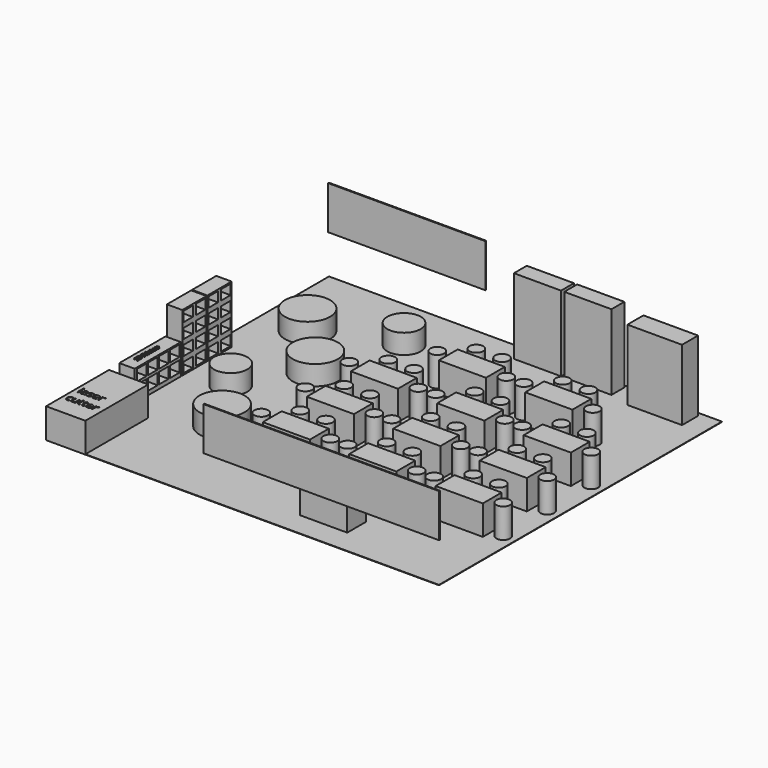
from build123d import *

# Parameters (mm, degrees)
F0_W          = 10000
F0_H          = 9000
F1_DEPTH      = 10
F2_W          = 1200
F2_H          = 600
F2_R          = 175
F3_DEPTH      = 750
F5_W          = 6000
F5_H          = 1100
F6_DEPTH      = 25
F8_W          = 1200
F8_H          = 410
F9_DEPTH      = 1920
F10_W         = 1390
F10_H         = 510
F11_DEPTH     = 1800
F12_W         = 4000
F12_H         = 1100
F13_DEPTH     = 25
F15_W         = 770
F15_H         = 1470
F15_W_2       = 298.1355935335
F15_H_2       = 253.6377906799
F16_DEPTH     = 390
F17_R         = 575
F17_R_2       = 425
F18_DEPTH     = 500
F19_W         = 1000
F19_H         = 2000
F19_W_2       = 23.0397869153
F19_H_2       = 215.8814716164
F20_DEPTH     = 750
F21_W         = 311.8368387222
F21_H         = 282.1381092072
F22_DEPTH     = 390
F23_TEXT_SIZE = 138.8888888889
F24_DEPTH     = 25


# Not quite as in the source:
# - Text() gives the source's letters only with a copy of the font that has no kerning and outlines rounded to 1/6400 em; it was checked with that copy


with BuildPart() as f1:
    # F0 (on Top) → F1 (new body)
    with BuildSketch(Plane.XY):
        Rectangle(F0_W, F0_H)
    extrude(amount=-F1_DEPTH)

    # F2 (on Top) → F3 (join)
    with BuildSketch(Plane.XY):
        with Locations((1572.2411870956, -3585.0810220754)):
            Rectangle(F2_W, F2_H)
        with Locations((3789.9301052094, -2043.914437294)):
            Rectangle(F2_W, F2_H)
        with Locations((2914.3524169922, -2047.3065376282)):
            Circle(F2_R)
        with Locations((4108.0131530762, -1479.732632637)):
            Circle(F2_R)
        with Locations((3458.5213661194, -1485.5839014053)):
            Circle(F2_R)
        with Locations((4681.4386844635, -2059.0091347694)):
            Circle(F2_R)
        with Locations((2914.3524169922, -647.3065376282)):
            Circle(F2_R)
        with Locations((4681.4386844635, -659.0091347694)):
            Circle(F2_R)
        with Locations((3789.9301052094, -643.914437294)):
            Rectangle(F2_W, F2_H)
        with Locations((3458.5213661194, -85.5839014053)):
            Circle(F2_R)
        with Locations((4108.0131530762, -79.732632637)):
            Circle(F2_R)
        with Locations((2914.3524169922, 752.6934623718)):
            Circle(F2_R)
        with Locations((4681.4386844635, 740.9908652306)):
            Circle(F2_R)
        with Locations((3789.9301052094, 756.085562706)):
            Rectangle(F2_W, F2_H)
        with Locations((3458.5213661194, 1314.4160985947)):
            Circle(F2_R)
        with Locations((4108.0131530762, 1320.267367363)):
            Circle(F2_R)
        with Locations((714.3524169922, -2047.3065376282)):
            Circle(F2_R)
        with Locations((2481.4386844635, -2059.0091347694)):
            Circle(F2_R)
        with Locations((1589.9301052094, -2043.914437294)):
            Rectangle(F2_W, F2_H)
        with Locations((1258.5213661194, -1485.5839014053)):
            Circle(F2_R)
        with Locations((1908.0131530762, -1479.732632637)):
            Circle(F2_R)
        with Locations((714.3524169922, -647.3065376282)):
            Circle(F2_R)
        with Locations((2481.4386844635, -659.0091347694)):
            Circle(F2_R)
        with Locations((1589.9301052094, -643.914437294)):
            Rectangle(F2_W, F2_H)
        with Locations((1258.5213661194, -85.5839014053)):
            Circle(F2_R)
        with Locations((1908.0131530762, -79.732632637)):
            Circle(F2_R)
        with Locations((714.3524169922, 752.6934623718)):
            Circle(F2_R)
        with Locations((2481.4386844635, 740.9908652306)):
            Circle(F2_R)
        with Locations((1589.9301052094, 756.085562706)):
            Rectangle(F2_W, F2_H)
        with Locations((1258.5213661194, 1314.4160985947)):
            Circle(F2_R)
        with Locations((1908.0131530762, 1320.267367363)):
            Circle(F2_R)
        with Locations((-1485.6475830078, -2047.3065376282)):
            Circle(F2_R)
        with Locations((281.4386844635, -2059.0091347694)):
            Circle(F2_R)
        with Locations((-610.0698947906, -2043.914437294)):
            Rectangle(F2_W, F2_H)
        with Locations((-941.4786338806, -1485.5839014053)):
            Circle(F2_R)
        with Locations((-291.9868469238, -1479.732632637)):
            Circle(F2_R)
        with Locations((-1485.6475830078, -647.3065376282)):
            Circle(F2_R)
        with Locations((281.4386844635, -659.0091347694)):
            Circle(F2_R)
        with Locations((-610.0698947906, -643.914437294)):
            Rectangle(F2_W, F2_H)
        with Locations((-941.4786338806, -85.5839014053)):
            Circle(F2_R)
        with Locations((-291.9868469238, -79.732632637)):
            Circle(F2_R)
        with Locations((-1485.6475830078, 752.6934623718)):
            Circle(F2_R)
        with Locations((281.4386844635, 740.9908652306)):
            Circle(F2_R)
        with Locations((-610.0698947906, 756.085562706)):
            Rectangle(F2_W, F2_H)
        with Locations((-941.4786338806, 1314.4160985947)):
            Circle(F2_R)
        with Locations((-291.9868469238, 1320.267367363)):
            Circle(F2_R)
        with Locations((1784.7433149815, 2214.4345091656)):
            Circle(F2_R)
        with Locations((3551.8295824528, 2202.7319120243)):
            Circle(F2_R)
        with Locations((2660.3210031986, 2217.8266094998)):
            Rectangle(F2_W, F2_H)
        with Locations((2328.9122641087, 2776.1571453884)):
            Circle(F2_R)
        with Locations((2978.4040510654, 2782.0084141567)):
            Circle(F2_R)
        with Locations((-415.2566850185, 2214.4345091656)):
            Circle(F2_R)
        with Locations((1351.8295824528, 2202.7319120243)):
            Circle(F2_R)
        with Locations((460.3210031986, 2217.8266094998)):
            Rectangle(F2_W, F2_H)
        with Locations((128.9122641087, 2776.1571453884)):
            Circle(F2_R)
        with Locations((778.4040510654, 2782.0084141567)):
            Circle(F2_R)
    extrude(amount=F3_DEPTH)

    # F8 (on Top) → F9 (join)
    with BuildSketch(Plane.XY):
        with Locations((686.8221908808, 4228.9738616641)):
            Rectangle(F8_W, F8_H)
        with Locations((1969.4395661354, 4228.5027503967)):
            Rectangle(F8_W, F8_H)
    extrude(amount=F9_DEPTH)

    # F10 (on Top) → F11 (join)
    with BuildSketch(Plane.XY):
        with Locations((3781.6548347473, 4139.8178529011)):
            Rectangle(F10_W, F10_H)
    extrude(amount=F11_DEPTH)

    # F15 (on offset) → F16 (join)
    with BuildSketch(Plane.YZ.offset(-5000)):
        with Locations((529.4889600399, 735)):
            Rectangle(F15_W, F15_H)
        with Locations((329.677836597, 165.8990240097)):
            Rectangle(F15_W_2, F15_H_2, mode=Mode.SUBTRACT)
        with Locations((729.677836597, 165.8990240097)):
            Rectangle(F15_W_2, F15_H_2, mode=Mode.SUBTRACT)
        with Locations((329.677836597, 545.8990240097)):
            Rectangle(F15_W_2, F15_H_2, mode=Mode.SUBTRACT)
        with Locations((729.677836597, 545.8990240097)):
            Rectangle(F15_W_2, F15_H_2, mode=Mode.SUBTRACT)
        with Locations((329.677836597, 925.8990240097)):
            Rectangle(F15_W_2, F15_H_2, mode=Mode.SUBTRACT)
        with Locations((729.677836597, 925.8990240097)):
            Rectangle(F15_W_2, F15_H_2, mode=Mode.SUBTRACT)
        with Locations((329.677836597, 1305.8990240097)):
            Rectangle(F15_W_2, F15_H_2, mode=Mode.SUBTRACT)
        with Locations((729.677836597, 1305.8990240097)):
            Rectangle(F15_W_2, F15_H_2, mode=Mode.SUBTRACT)
        with Locations((-270.5110399601, 735)):
            Rectangle(F15_W, F15_H)
        with Locations((-470.322163403, 165.8990240097)):
            Rectangle(F15_W_2, F15_H_2, mode=Mode.SUBTRACT)
        with Locations((-70.322163403, 165.8990240097)):
            Rectangle(F15_W_2, F15_H_2, mode=Mode.SUBTRACT)
        with Locations((-470.322163403, 545.8990240097)):
            Rectangle(F15_W_2, F15_H_2, mode=Mode.SUBTRACT)
        with Locations((-70.322163403, 545.8990240097)):
            Rectangle(F15_W_2, F15_H_2, mode=Mode.SUBTRACT)
        with Locations((-470.322163403, 925.8990240097)):
            Rectangle(F15_W_2, F15_H_2, mode=Mode.SUBTRACT)
        with Locations((-70.322163403, 925.8990240097)):
            Rectangle(F15_W_2, F15_H_2, mode=Mode.SUBTRACT)
        with Locations((-470.322163403, 1305.8990240097)):
            Rectangle(F15_W_2, F15_H_2, mode=Mode.SUBTRACT)
        with Locations((-70.322163403, 1305.8990240097)):
            Rectangle(F15_W_2, F15_H_2, mode=Mode.SUBTRACT)
    extrude(amount=F16_DEPTH)

    # F17 (on Top) → F18 (join)
    with BuildSketch(Plane.XY):
        with Locations((-3872.6794719696, 2408.0123901367)):
            Circle(F17_R)
        with Locations((-2614.8862838745, 1084.0193033218)):
            Circle(F17_R)
        with Locations((-2631.4361095428, -1861.8651628494)):
            Circle(F17_R)
        with Locations((-3591.3310050964, -388.9229595661)):
            Circle(F17_R_2)
        with Locations((-1985.9894514084, 3119.6584701538)):
            Circle(F17_R_2)
    extrude(amount=F18_DEPTH)

    # F19 (on face) → F20 (join)
    with BuildSketch(Plane.XY):
        with Locations((-4500, -3500)):
            Rectangle(F19_W, F19_H)
        with BuildLine():
            add(Edge.make_bspline(
                [(-4797.4227787473, -4022.5041243538), (-4812.6494587318, -4030.4504092436), (-4835.8224236061, -4030.4504092436)],
                knots=[0, 0, 0, 1, 1, 1], degree=2))
            add(Edge.make_bspline(
                [(-4835.8224236061, -4030.4504092436), (-4868.8505574499, -4030.4504092436), (-4886.9627598804, -4010.1185741624)],
                knots=[0, 0, 0, 1, 1, 1], degree=2))
            add(Edge.make_bspline(
                [(-4886.9627598804, -4010.1185741624), (-4905.0749623109, -3989.7867390811), (-4905.0749623109, -3952.5856958537)],
                knots=[0, 0, 0, 1, 1, 1], degree=2))
            add(Edge.make_bspline(
                [(-4905.0749623109, -3952.5856958537), (-4905.0749623109, -3914.452406913), (-4886.6742076358, -3893.6322526486)],
                knots=[0, 0, 0, 1, 1, 1], degree=2))
            add(Edge.make_bspline(
                [(-4886.6742076358, -3893.6322526486), (-4868.2734529607, -3872.8120983841), (-4834.3130734035, -3872.8120983841)],
                knots=[0, 0, 0, 1, 1, 1], degree=2))
            add(Edge.make_bspline(
                [(-4834.3130734035, -3872.8120983841), (-4823.3480881086, -3872.8120983841), (-4812.3831028137, -3875.1871053204)],
                knots=[0, 0, 0, 1, 1, 1], degree=2))
            add(Edge.make_bspline(
                [(-4812.3831028137, -3875.1871053204), (-4801.4181175187, -3877.5621122568), (-4795.2031460965, -3880.7583832739)],
                knots=[0, 0, 0, 1, 1, 1], degree=2))
            Line((-4795.2031460965, -3880.7583832739), (-4802.2615779261, -3900.291150601))
            add(Edge.make_bspline(
                [(-4802.2615779261, -3900.291150601), (-4809.8971142448, -3897.2280575429), (-4818.908822807, -3895.2303881571)],
                knots=[0, 0, 0, 1, 1, 1], degree=2))
            add(Edge.make_bspline(
                [(-4818.908822807, -3895.2303881571), (-4827.9205313693, -3893.2327187714), (-4834.8457852397, -3893.2327187714)],
                knots=[0, 0, 0, 1, 1, 1], degree=2))
            add(Edge.make_bspline(
                [(-4834.8457852397, -3893.2327187714), (-4881.1917149884, -3893.2327187714), (-4881.1917149884, -3952.3193399356)],
                knots=[0, 0, 0, 1, 1, 1], degree=2))
            add(Edge.make_bspline(
                [(-4881.1917149884, -3952.3193399356), (-4881.1917149884, -3980.3311039887), (-4869.8937847958, -3995.3136243815)],
                knots=[0, 0, 0, 1, 1, 1], degree=2))
            add(Edge.make_bspline(
                [(-4869.8937847958, -3995.3136243815), (-4858.5958546033, -4010.2961447744), (-4836.3995280953, -4010.2961447744)],
                knots=[0, 0, 0, 1, 1, 1], degree=2))
            add(Edge.make_bspline(
                [(-4836.3995280953, -4010.2961447744), (-4817.3994726045, -4010.2961447744), (-4797.4227787473, -4002.1278966195)],
                knots=[0, 0, 0, 1, 1, 1], degree=2))
            Line((-4797.4227787473, -4002.1278966195), (-4797.4227787473, -4022.5041243538))
        make_face(mode=Mode.SUBTRACT)
        with BuildLine():
            Line((-4762.974080007, -3875.6088355241), (-4739.6679371736, -3875.6088355241))
            Line((-4739.6679371736, -3875.6088355241), (-4739.6679371736, -3974.2493105255))
            add(Edge.make_bspline(
                [(-4739.6679371736, -3974.2493105255), (-4739.6679371736, -3992.8498321392), (-4731.2111367741, -4001.9947186604)],
                knots=[0, 0, 0, 1, 1, 1], degree=2))
            add(Edge.make_bspline(
                [(-4731.2111367741, -4001.9947186604), (-4722.7543363745, -4011.1396051817), (-4704.7309192501, -4011.1396051817)],
                knots=[0, 0, 0, 1, 1, 1], degree=2))
            add(Edge.make_bspline(
                [(-4704.7309192501, -4011.1396051817), (-4680.8476719275, -4011.1396051817), (-4669.8382939795, -3998.1103615215)],
                knots=[0, 0, 0, 1, 1, 1], degree=2))
            add(Edge.make_bspline(
                [(-4669.8382939795, -3998.1103615215), (-4658.8289160316, -3985.0811178614), (-4658.8289160316, -3955.5156109528)],
                knots=[0, 0, 0, 1, 1, 1], degree=2))
            Line((-4658.8289160316, -3955.5156109528), (-4658.8289160316, -3875.6088355241))
            Line((-4658.8289160316, -3875.6088355241), (-4635.7891291163, -3875.6088355241))
            Line((-4635.7891291163, -3875.6088355241), (-4635.7891291163, -4027.6536721036))
            Line((-4635.7891291163, -4027.6536721036), (-4654.7891846071, -4027.6536721036))
            Line((-4654.7891846071, -4027.6536721036), (-4658.1186335833, -4007.2774443693))
            Line((-4658.1186335833, -4007.2774443693), (-4659.3616278678, -4007.2774443693))
            add(Edge.make_bspline(
                [(-4659.3616278678, -4007.2774443693), (-4666.4200596973, -4018.5087855824), (-4678.9831805008, -4024.479597413)],
                knots=[0, 0, 0, 1, 1, 1], degree=2))
            add(Edge.make_bspline(
                [(-4678.9831805008, -4024.479597413), (-4691.5463013043, -4030.4504092436), (-4707.6608343491, -4030.4504092436)],
                knots=[0, 0, 0, 1, 1, 1], degree=2))
            add(Edge.make_bspline(
                [(-4707.6608343491, -4030.4504092436), (-4735.4062424841, -4030.4504092436), (-4749.1901612455, -4017.2657912979)],
                knots=[0, 0, 0, 1, 1, 1], degree=2))
            add(Edge.make_bspline(
                [(-4749.1901612455, -4017.2657912979), (-4762.974080007, -4004.0811733522), (-4762.974080007, -3975.0927709328)],
                knots=[0, 0, 0, 1, 1, 1], degree=2))
            Line((-4762.974080007, -3975.0927709328), (-4762.974080007, -3875.6088355241))
        make_face(mode=Mode.SUBTRACT)
        with BuildLine():
            add(Edge.make_bspline(
                [(-4295.8745849734, -4028.1419912868), (-4306.7507849623, -4030.4504092436), (-4322.1550355588, -4030.4504092436)],
                knots=[0, 0, 0, 1, 1, 1], degree=2))
            add(Edge.make_bspline(
                [(-4322.1550355588, -4030.4504092436), (-4355.8490591979, -4030.4504092436), (-4375.3596301984, -4009.8966108973)],
                knots=[0, 0, 0, 1, 1, 1], degree=2))
            add(Edge.make_bspline(
                [(-4375.3596301984, -4009.8966108973), (-4394.8702011989, -3989.3428125509), (-4394.8702011989, -3952.8964444248)],
                knots=[0, 0, 0, 1, 1, 1], degree=2))
            add(Edge.make_bspline(
                [(-4394.8702011989, -3952.8964444248), (-4394.8702011989, -3916.0949350746), (-4376.7579987684, -3894.4535167294)],
                knots=[0, 0, 0, 1, 1, 1], degree=2))
            add(Edge.make_bspline(
                [(-4376.7579987684, -3894.4535167294), (-4358.6457963379, -3872.8120983841), (-4328.1036510629, -3872.8120983841)],
                knots=[0, 0, 0, 1, 1, 1], degree=2))
            add(Edge.make_bspline(
                [(-4328.1036510629, -3872.8120983841), (-4299.5591751737, -3872.8120983841), (-4282.9119302927, -3891.6123869363)],
                knots=[0, 0, 0, 1, 1, 1], degree=2))
            add(Edge.make_bspline(
                [(-4282.9119302927, -3891.6123869363), (-4266.2646854118, -3910.4126754886), (-4266.2646854118, -3941.2211766816)],
                knots=[0, 0, 0, 1, 1, 1], degree=2))
            Line((-4266.2646854118, -3941.2211766816), (-4266.2646854118, -3955.7819668709))
            Line((-4266.2646854118, -3955.7819668709), (-4370.9869538763, -3955.7819668709))
            add(Edge.make_bspline(
                [(-4370.9869538763, -3955.7819668709), (-4370.2766714281, -3982.5507366395), (-4357.4471947065, -3996.4234407069)],
                knots=[0, 0, 0, 1, 1, 1], degree=2))
            add(Edge.make_bspline(
                [(-4357.4471947065, -3996.4234407069), (-4344.6177179849, -4010.2961447744), (-4321.3115751515, -4010.2961447744)],
                knots=[0, 0, 0, 1, 1, 1], degree=2))
            add(Edge.make_bspline(
                [(-4321.3115751515, -4010.2961447744), (-4296.7624380337, -4010.2961447744), (-4272.7904054051, -4000.0414419277)],
                knots=[0, 0, 0, 1, 1, 1], degree=2))
            Line((-4272.7904054051, -4000.0414419277), (-4272.7904054051, -4020.5952402741))
            add(Edge.make_bspline(
                [(-4272.7904054051, -4020.5952402741), (-4284.9983849845, -4025.83357333), (-4295.8745849734, -4028.1419912868)],
                knots=[0, 0, 0, 1, 1, 1], degree=2))
        make_face(mode=Mode.SUBTRACT)
        with BuildLine():
            add(Edge.make_bspline(
                [(-4183.8275287612, -3880.8693649065), (-4171.8859050999, -3872.8120983841), (-4157.5914708288, -3872.8120983841)],
                knots=[0, 0, 0, 1, 1, 1], degree=2))
            add(Edge.make_bspline(
                [(-4157.5914708288, -3872.8120983841), (-4147.4699459411, -3872.8120983841), (-4139.4348757453, -3874.4990191987)],
                knots=[0, 0, 0, 1, 1, 1], degree=2))
            Line((-4139.4348757453, -3874.4990191987), (-4142.6311467624, -3895.8518852994))
            add(Edge.make_bspline(
                [(-4142.6311467624, -3895.8518852994), (-4152.0423892018, -3893.7654306076), (-4159.2783916434, -3893.7654306076)],
                knots=[0, 0, 0, 1, 1, 1], degree=2))
            add(Edge.make_bspline(
                [(-4159.2783916434, -3893.7654306076), (-4177.745735298, -3893.7654306076), (-4190.8415679377, -3908.7479510005)],
                knots=[0, 0, 0, 1, 1, 1], degree=2))
            add(Edge.make_bspline(
                [(-4190.8415679377, -3908.7479510005), (-4203.9374005774, -3923.7304713934), (-4203.9374005774, -3946.0599758604)],
                knots=[0, 0, 0, 1, 1, 1], degree=2))
            Line((-4203.9374005774, -3946.0599758604), (-4203.9374005774, -4027.6536721036))
            Line((-4203.9374005774, -4027.6536721036), (-4226.9771874927, -4027.6536721036))
            Line((-4226.9771874927, -4027.6536721036), (-4226.9771874927, -3875.6088355241))
            Line((-4226.9771874927, -3875.6088355241), (-4207.9771320019, -3875.6088355241))
            Line((-4207.9771320019, -3875.6088355241), (-4205.3135728209, -3903.7537775362))
            Line((-4205.3135728209, -3903.7537775362), (-4204.2037564955, -3903.7537775362))
            add(Edge.make_bspline(
                [(-4204.2037564955, -3903.7537775362), (-4195.7691524225, -3888.9266314289), (-4183.8275287612, -3880.8693649065)],
                knots=[0, 0, 0, 1, 1, 1], degree=2))
        make_face(mode=Mode.SUBTRACT)
        with BuildLine():
            add(Edge.make_bspline(
                [(-4555.7491757286, -4004.0589770257), (-4549.2234557353, -4011.4059610998), (-4537.8589365632, -4011.4059610998)],
                knots=[0, 0, 0, 1, 1, 1], degree=2))
            add(Edge.make_bspline(
                [(-4537.8589365632, -4011.4059610998), (-4531.732750447, -4011.4059610998), (-4526.050490861, -4010.5181080395)],
                knots=[0, 0, 0, 1, 1, 1], degree=2))
            add(Edge.make_bspline(
                [(-4526.050490861, -4010.5181080395), (-4520.3682312749, -4009.6302549792), (-4517.0387822987, -4008.6536166128)],
                knots=[0, 0, 0, 1, 1, 1], degree=2))
            Line((-4517.0387822987, -4008.6536166128), (-4517.0387822987, -4026.2774998602))
            add(Edge.make_bspline(
                [(-4517.0387822987, -4026.2774998602), (-4520.7677651521, -4028.0532059808), (-4528.0481602467, -4029.2518076122)],
                knots=[0, 0, 0, 1, 1, 1], degree=2))
            add(Edge.make_bspline(
                [(-4528.0481602467, -4029.2518076122), (-4535.3285553413, -4030.4504092436), (-4541.1883855394, -4030.4504092436)],
                knots=[0, 0, 0, 1, 1, 1], degree=2))
            add(Edge.make_bspline(
                [(-4541.1883855394, -4030.4504092436), (-4585.2702899842, -4030.4504092436), (-4585.2702899842, -3983.971301536)],
                knots=[0, 0, 0, 1, 1, 1], degree=2))
            Line((-4585.2702899842, -3983.971301536), (-4585.2702899842, -3893.4990746895))
            Line((-4585.2702899842, -3893.4990746895), (-4607.067082615, -3893.4990746895))
            Line((-4607.067082615, -3893.4990746895), (-4607.067082615, -3882.4009114355))
            Line((-4607.067082615, -3882.4009114355), (-4585.2702899842, -3872.8120983841))
            Line((-4585.2702899842, -3872.8120983841), (-4575.5926916267, -3840.3610690295))
            Line((-4575.5926916267, -3840.3610690295), (-4562.274895722, -3840.3610690295))
            Line((-4562.274895722, -3840.3610690295), (-4562.274895722, -3875.6088355241))
            Line((-4562.274895722, -3875.6088355241), (-4518.1485986241, -3875.6088355241))
            Line((-4518.1485986241, -3875.6088355241), (-4518.1485986241, -3893.4990746895))
            Line((-4518.1485986241, -3893.4990746895), (-4562.274895722, -3893.4990746895))
            Line((-4562.274895722, -3893.4990746895), (-4562.274895722, -3982.9946631696))
            add(Edge.make_bspline(
                [(-4562.274895722, -3982.9946631696), (-4562.274895722, -3996.7119929515), (-4555.7491757286, -4004.0589770257)],
                knots=[0, 0, 0, 1, 1, 1], degree=2))
        make_face(mode=Mode.SUBTRACT)
        with BuildLine():
            add(Edge.make_bspline(
                [(-4455.4661725656, -4004.0589770257), (-4448.9404525723, -4011.4059610998), (-4437.5759334002, -4011.4059610998)],
                knots=[0, 0, 0, 1, 1, 1], degree=2))
            add(Edge.make_bspline(
                [(-4437.5759334002, -4011.4059610998), (-4431.449747284, -4011.4059610998), (-4425.767487698, -4010.5181080395)],
                knots=[0, 0, 0, 1, 1, 1], degree=2))
            add(Edge.make_bspline(
                [(-4425.767487698, -4010.5181080395), (-4420.0852281119, -4009.6302549792), (-4416.7557791358, -4008.6536166128)],
                knots=[0, 0, 0, 1, 1, 1], degree=2))
            Line((-4416.7557791358, -4008.6536166128), (-4416.7557791358, -4026.2774998602))
            add(Edge.make_bspline(
                [(-4416.7557791358, -4026.2774998602), (-4420.4847619891, -4028.0532059808), (-4427.7651570837, -4029.2518076122)],
                knots=[0, 0, 0, 1, 1, 1], degree=2))
            add(Edge.make_bspline(
                [(-4427.7651570837, -4029.2518076122), (-4435.0455521783, -4030.4504092436), (-4440.9053823764, -4030.4504092436)],
                knots=[0, 0, 0, 1, 1, 1], degree=2))
            add(Edge.make_bspline(
                [(-4440.9053823764, -4030.4504092436), (-4484.9872868212, -4030.4504092436), (-4484.9872868212, -3983.971301536)],
                knots=[0, 0, 0, 1, 1, 1], degree=2))
            Line((-4484.9872868212, -3983.971301536), (-4484.9872868212, -3893.4990746895))
            Line((-4484.9872868212, -3893.4990746895), (-4506.784079452, -3893.4990746895))
            Line((-4506.784079452, -3893.4990746895), (-4506.784079452, -3882.4009114355))
            Line((-4506.784079452, -3882.4009114355), (-4484.9872868212, -3872.8120983841))
            Line((-4484.9872868212, -3872.8120983841), (-4475.3096884638, -3840.3610690295))
            Line((-4475.3096884638, -3840.3610690295), (-4461.991892559, -3840.3610690295))
            Line((-4461.991892559, -3840.3610690295), (-4461.991892559, -3875.6088355241))
            Line((-4461.991892559, -3875.6088355241), (-4417.8655954611, -3875.6088355241))
            Line((-4417.8655954611, -3875.6088355241), (-4417.8655954611, -3893.4990746895))
            Line((-4417.8655954611, -3893.4990746895), (-4461.991892559, -3893.4990746895))
            Line((-4461.991892559, -3893.4990746895), (-4461.991892559, -3982.9946631696))
            add(Edge.make_bspline(
                [(-4461.991892559, -3982.9946631696), (-4461.991892559, -3996.7119929515), (-4455.4661725656, -4004.0589770257)],
                knots=[0, 0, 0, 1, 1, 1], degree=2))
        make_face(mode=Mode.SUBTRACT)
        with Locations((-4885.0760721273, -3533.3192844448)):
            Rectangle(F19_W_2, F19_H_2, mode=Mode.SUBTRACT)
        with BuildLine():
            Line((-4714.1421616894, -3641.260020253), (-4731.2333331006, -3641.260020253))
            Line((-4731.2333331006, -3641.260020253), (-4735.8057763612, -3619.5964055813))
            Line((-4735.8057763612, -3619.5964055813), (-4736.9155926866, -3619.5964055813))
            add(Edge.make_bspline(
                [(-4736.9155926866, -3619.5964055813), (-4748.2801118587, -3633.8908398524), (-4759.5780420512, -3638.9737986227)],
                knots=[0, 0, 0, 1, 1, 1], degree=2))
            add(Edge.make_bspline(
                [(-4759.5780420512, -3638.9737986227), (-4770.8759722438, -3644.056757393), (-4787.8339656959, -3644.056757393)],
                knots=[0, 0, 0, 1, 1, 1], degree=2))
            add(Edge.make_bspline(
                [(-4787.8339656959, -3644.056757393), (-4810.429826081, -3644.056757393), (-4823.2593028026, -3632.3814896498)],
                knots=[0, 0, 0, 1, 1, 1], degree=2))
            add(Edge.make_bspline(
                [(-4823.2593028026, -3632.3814896498), (-4836.0887795242, -3620.7062219067), (-4836.0887795242, -3599.2201778469)],
                knots=[0, 0, 0, 1, 1, 1], degree=2))
            add(Edge.make_bspline(
                [(-4836.0887795242, -3599.2201778469), (-4836.0887795242, -3553.1849966694), (-4762.4413681708, -3550.9653640186)],
                knots=[0, 0, 0, 1, 1, 1], degree=2))
            Line((-4762.4413681708, -3550.9653640186), (-4736.6492367685, -3550.1219036113))
            Line((-4736.6492367685, -3550.1219036113), (-4736.6492367685, -3540.6662685189))
            add(Edge.make_bspline(
                [(-4736.6492367685, -3540.6662685189), (-4736.6492367685, -3522.7760293535), (-4744.3291657403, -3514.2526399745)],
                knots=[0, 0, 0, 1, 1, 1], degree=2))
            add(Edge.make_bspline(
                [(-4744.3291657403, -3514.2526399745), (-4752.009094712, -3505.7292505954), (-4768.9670881641, -3505.7292505954)],
                knots=[0, 0, 0, 1, 1, 1], degree=2))
            add(Edge.make_bspline(
                [(-4768.9670881641, -3505.7292505954), (-4787.9671436549, -3505.7292505954), (-4811.9391762835, -3517.3601256856)],
                knots=[0, 0, 0, 1, 1, 1], degree=2))
            Line((-4811.9391762835, -3517.3601256856), (-4819.0420007661, -3499.7362424383))
            add(Edge.make_bspline(
                [(-4819.0420007661, -3499.7362424383), (-4807.810659553, -3493.6544489751), (-4794.4262746687, -3490.1918220398)],
                knots=[0, 0, 0, 1, 1, 1], degree=2))
            add(Edge.make_bspline(
                [(-4794.4262746687, -3490.1918220398), (-4781.0418897844, -3486.7291951046), (-4767.5465232676, -3486.7291951046)],
                knots=[0, 0, 0, 1, 1, 1], degree=2))
            add(Edge.make_bspline(
                [(-4767.5465232676, -3486.7291951046), (-4740.3782196218, -3486.7291951046), (-4727.2601906556, -3498.7818003984)],
                knots=[0, 0, 0, 1, 1, 1], degree=2))
            add(Edge.make_bspline(
                [(-4727.2601906556, -3498.7818003984), (-4714.1421616894, -3510.8344056922), (-4714.1421616894, -3537.4699975018)],
                knots=[0, 0, 0, 1, 1, 1], degree=2))
            Line((-4714.1421616894, -3537.4699975018), (-4714.1421616894, -3641.260020253))
        make_face(mode=Mode.SUBTRACT)
        with BuildLine():
            add(Edge.make_bspline(
                [(-4578.1674655017, -3574.6710407291), (-4568.6674377562, -3584.6593876577), (-4568.6674377562, -3599.7972823362)],
                knots=[0, 0, 0, 1, 1, 1], degree=2))
            add(Edge.make_bspline(
                [(-4568.6674377562, -3599.7972823362), (-4568.6674377562, -3621.0169704778), (-4584.4712222299, -3632.5368639354)],
                knots=[0, 0, 0, 1, 1, 1], degree=2))
            add(Edge.make_bspline(
                [(-4584.4712222299, -3632.5368639354), (-4600.2750067036, -3644.056757393), (-4628.8638752458, -3644.056757393)],
                knots=[0, 0, 0, 1, 1, 1], degree=2))
            add(Edge.make_bspline(
                [(-4628.8638752458, -3644.056757393), (-4659.0952719497, -3644.056757393), (-4676.0088727488, -3634.4679443416)],
                knots=[0, 0, 0, 1, 1, 1], degree=2))
            Line((-4676.0088727488, -3634.4679443416), (-4676.0088727488, -3613.1150782409))
            add(Edge.make_bspline(
                [(-4676.0088727488, -3613.1150782409), (-4665.0438874538, -3618.6641598679), (-4652.5029629768, -3621.8382345586)],
                knots=[0, 0, 0, 1, 1, 1], degree=2))
            add(Edge.make_bspline(
                [(-4652.5029629768, -3621.8382345586), (-4639.9620384998, -3625.0123092492), (-4628.2867707566, -3625.0123092492)],
                knots=[0, 0, 0, 1, 1, 1], degree=2))
            add(Edge.make_bspline(
                [(-4628.2867707566, -3625.0123092492), (-4610.2633536322, -3625.0123092492), (-4600.5635589482, -3619.2634606836)],
                knots=[0, 0, 0, 1, 1, 1], degree=2))
            add(Edge.make_bspline(
                [(-4600.5635589482, -3619.2634606836), (-4590.8637642642, -3613.5146121181), (-4590.8637642642, -3601.7061664158)],
                knots=[0, 0, 0, 1, 1, 1], degree=2))
            add(Edge.make_bspline(
                [(-4590.8637642642, -3601.7061664158), (-4590.8637642642, -3592.8276358127), (-4598.543693236, -3586.5238790844)],
                knots=[0, 0, 0, 1, 1, 1], degree=2))
            add(Edge.make_bspline(
                [(-4598.543693236, -3586.5238790844), (-4606.2236222077, -3580.2201223561), (-4628.5975193277, -3571.607947671)],
                knots=[0, 0, 0, 1, 1, 1], degree=2))
            add(Edge.make_bspline(
                [(-4628.5975193277, -3571.607947671), (-4649.8172074694, -3563.7060554342), (-4658.7623270521, -3557.8018325831)],
                knots=[0, 0, 0, 1, 1, 1], degree=2))
            add(Edge.make_bspline(
                [(-4658.7623270521, -3557.8018325831), (-4667.7074466348, -3551.897609732), (-4672.0801229568, -3544.4174476988)],
                knots=[0, 0, 0, 1, 1, 1], degree=2))
            add(Edge.make_bspline(
                [(-4672.0801229568, -3544.4174476988), (-4676.4527992789, -3536.9372856656), (-4676.4527992789, -3526.5494048599)],
                knots=[0, 0, 0, 1, 1, 1], degree=2))
            add(Edge.make_bspline(
                [(-4676.4527992789, -3526.5494048599), (-4676.4527992789, -3507.9488832462), (-4661.3149046005, -3497.1836648898)],
                knots=[0, 0, 0, 1, 1, 1], degree=2))
            add(Edge.make_bspline(
                [(-4661.3149046005, -3497.1836648898), (-4646.1770099221, -3486.4184465335), (-4619.8521666836, -3486.4184465335)],
                knots=[0, 0, 0, 1, 1, 1], degree=2))
            add(Edge.make_bspline(
                [(-4619.8521666836, -3486.4184465335), (-4595.3030295658, -3486.4184465335), (-4571.8193161204, -3496.4067934621)],
                knots=[0, 0, 0, 1, 1, 1], degree=2))
            Line((-4571.8193161204, -3496.4067934621), (-4580.0319569283, -3515.1404930348))
            add(Edge.make_bspline(
                [(-4580.0319569283, -3515.1404930348), (-4602.8941732315, -3505.7292505954), (-4621.4946948452, -3505.7292505954)],
                knots=[0, 0, 0, 1, 1, 1], degree=2))
            add(Edge.make_bspline(
                [(-4621.4946948452, -3505.7292505954), (-4637.8755838081, -3505.7292505954), (-4646.1992062486, -3510.8566020187)],
                knots=[0, 0, 0, 1, 1, 1], degree=2))
            add(Edge.make_bspline(
                [(-4646.1992062486, -3510.8566020187), (-4654.522828689, -3515.9839534421), (-4654.522828689, -3524.9956620043)],
                knots=[0, 0, 0, 1, 1, 1], degree=2))
            add(Edge.make_bspline(
                [(-4654.522828689, -3524.9956620043), (-4654.522828689, -3531.1218481205), (-4651.3931466514, -3535.4057391366)],
                knots=[0, 0, 0, 1, 1, 1], degree=2))
            add(Edge.make_bspline(
                [(-4651.3931466514, -3535.4057391366), (-4648.2634646138, -3539.6896301526), (-4641.3382107433, -3543.5739872915)],
                knots=[0, 0, 0, 1, 1, 1], degree=2))
            add(Edge.make_bspline(
                [(-4641.3382107433, -3543.5739872915), (-4634.4129568728, -3547.4583444304), (-4614.7026189338, -3554.827524831)],
                knots=[0, 0, 0, 1, 1, 1], degree=2))
            add(Edge.make_bspline(
                [(-4614.7026189338, -3554.827524831), (-4587.6674932471, -3564.6826938006), (-4578.1674655017, -3574.6710407291)],
                knots=[0, 0, 0, 1, 1, 1], degree=2))
        make_face(mode=Mode.SUBTRACT)
        with BuildLine():
            add(Edge.make_bspline(
                [(-4440.6834191113, -3641.7483394362), (-4451.5596191002, -3644.056757393), (-4466.9638696968, -3644.056757393)],
                knots=[0, 0, 0, 1, 1, 1], degree=2))
            add(Edge.make_bspline(
                [(-4466.9638696968, -3644.056757393), (-4500.6578933359, -3644.056757393), (-4520.1684643363, -3623.5029590467)],
                knots=[0, 0, 0, 1, 1, 1], degree=2))
            add(Edge.make_bspline(
                [(-4520.1684643363, -3623.5029590467), (-4539.6790353368, -3602.9491607003), (-4539.6790353368, -3566.5027925742)],
                knots=[0, 0, 0, 1, 1, 1], degree=2))
            add(Edge.make_bspline(
                [(-4539.6790353368, -3566.5027925742), (-4539.6790353368, -3529.701283224), (-4521.5668329064, -3508.0598648787)],
                knots=[0, 0, 0, 1, 1, 1], degree=2))
            add(Edge.make_bspline(
                [(-4521.5668329064, -3508.0598648787), (-4503.4546304759, -3486.4184465335), (-4472.9124852009, -3486.4184465335)],
                knots=[0, 0, 0, 1, 1, 1], degree=2))
            add(Edge.make_bspline(
                [(-4472.9124852009, -3486.4184465335), (-4444.3680093117, -3486.4184465335), (-4427.7207644307, -3505.2187350857)],
                knots=[0, 0, 0, 1, 1, 1], degree=2))
            add(Edge.make_bspline(
                [(-4427.7207644307, -3505.2187350857), (-4411.0735195497, -3524.019023638), (-4411.0735195497, -3554.827524831)],
                knots=[0, 0, 0, 1, 1, 1], degree=2))
            Line((-4411.0735195497, -3554.827524831), (-4411.0735195497, -3569.3883150202))
            Line((-4411.0735195497, -3569.3883150202), (-4515.7957880143, -3569.3883150202))
            add(Edge.make_bspline(
                [(-4515.7957880143, -3569.3883150202), (-4515.085505566, -3596.1570847888), (-4502.2560288444, -3610.0297888563)],
                knots=[0, 0, 0, 1, 1, 1], degree=2))
            add(Edge.make_bspline(
                [(-4502.2560288444, -3610.0297888563), (-4489.4265521228, -3623.9024929238), (-4466.1204092895, -3623.9024929238)],
                knots=[0, 0, 0, 1, 1, 1], degree=2))
            add(Edge.make_bspline(
                [(-4466.1204092895, -3623.9024929238), (-4441.5712721717, -3623.9024929238), (-4417.5992395431, -3613.6477900771)],
                knots=[0, 0, 0, 1, 1, 1], degree=2))
            Line((-4417.5992395431, -3613.6477900771), (-4417.5992395431, -3634.2015884235))
            add(Edge.make_bspline(
                [(-4417.5992395431, -3634.2015884235), (-4429.8072191224, -3639.4399214794), (-4440.6834191113, -3641.7483394362)],
                knots=[0, 0, 0, 1, 1, 1], degree=2))
        make_face(mode=Mode.SUBTRACT)
        with BuildLine():
            add(Edge.make_bspline(
                [(-4328.6363628991, -3494.4757130559), (-4316.6947392379, -3486.4184465335), (-4302.4003049667, -3486.4184465335)],
                knots=[0, 0, 0, 1, 1, 1], degree=2))
            add(Edge.make_bspline(
                [(-4302.4003049667, -3486.4184465335), (-4292.2787800791, -3486.4184465335), (-4284.2437098832, -3488.1053673481)],
                knots=[0, 0, 0, 1, 1, 1], degree=2))
            Line((-4284.2437098832, -3488.1053673481), (-4287.4399809004, -3509.4582334487))
            add(Edge.make_bspline(
                [(-4287.4399809004, -3509.4582334487), (-4296.8512233397, -3507.371778757), (-4304.0872257813, -3507.371778757)],
                knots=[0, 0, 0, 1, 1, 1], degree=2))
            add(Edge.make_bspline(
                [(-4304.0872257813, -3507.371778757), (-4322.554569436, -3507.371778757), (-4335.6504020757, -3522.3542991499)],
                knots=[0, 0, 0, 1, 1, 1], degree=2))
            add(Edge.make_bspline(
                [(-4335.6504020757, -3522.3542991499), (-4348.7462347154, -3537.3368195427), (-4348.7462347154, -3559.6663240098)],
                knots=[0, 0, 0, 1, 1, 1], degree=2))
            Line((-4348.7462347154, -3559.6663240098), (-4348.7462347154, -3641.260020253))
            Line((-4348.7462347154, -3641.260020253), (-4371.7860216306, -3641.260020253))
            Line((-4371.7860216306, -3641.260020253), (-4371.7860216306, -3489.2151836735))
            Line((-4371.7860216306, -3489.2151836735), (-4352.7859661398, -3489.2151836735))
            Line((-4352.7859661398, -3489.2151836735), (-4350.1224069588, -3517.3601256856))
            Line((-4350.1224069588, -3517.3601256856), (-4349.0125906334, -3517.3601256856))
            add(Edge.make_bspline(
                [(-4349.0125906334, -3517.3601256856), (-4340.5779865604, -3502.5329795783), (-4328.6363628991, -3494.4757130559)],
                knots=[0, 0, 0, 1, 1, 1], degree=2))
        make_face(mode=Mode.SUBTRACT)
    extrude(amount=F20_DEPTH)

    # F21 (on offset) → F22 (join)
    with BuildSketch(Plane.YZ.offset(-5000)):
        Polygon((-700, 420), (-700, 770), (-1050, 770), (-1050, 734.7841262817), (-739.9241924286, 734.7841262817), (-739.9241924286, 452.6460170746), (-1050, 452.6460170746), (-1050, 420), (-1050, 384.7841262817), (-739.9241924286, 384.7841262817), (-739.9241924286, 102.6460170746), (-1050, 102.6460170746), (-1050, 0), (-700, 0), align=None)
        Polygon((-1050, 734.7841262817), (-1050, 770), (-1400, 770), (-1400, 734.7841262817), (-1089.9241924286, 734.7841262817), (-1089.9241924286, 452.6460170746), (-1400, 452.6460170746), (-1400, 420), (-1400, 384.7841262817), (-1089.9241924286, 384.7841262817), (-1089.9241924286, 102.6460170746), (-1400, 102.6460170746), (-1400, 0), (-1050, 0), (-1050, 102.6460170746), (-1051.7610311508, 102.6460170746), (-1051.7610311508, 384.7841262817), (-1050, 384.7841262817), (-1050, 420), (-1050, 452.6460170746), (-1051.7610311508, 452.6460170746), (-1051.7610311508, 734.7841262817), align=None)
        Polygon((-1400, 734.7841262817), (-1400, 770), (-1750, 770), (-1750, 734.7841262817), (-1439.9241924286, 734.7841262817), (-1439.9241924286, 452.6460170746), (-1750, 452.6460170746), (-1750, 420), (-1750, 384.7841262817), (-1439.9241924286, 384.7841262817), (-1439.9241924286, 102.6460170746), (-1750, 102.6460170746), (-1750, 0), (-1400, 0), (-1400, 102.6460170746), (-1401.7610311508, 102.6460170746), (-1401.7610311508, 384.7841262817), (-1400, 384.7841262817), (-1400, 420), (-1400, 452.6460170746), (-1401.7610311508, 452.6460170746), (-1401.7610311508, 734.7841262817), align=None)
        Polygon((-1750, 734.7841262817), (-1750, 770), (-2170, 770), (-2170, 0), (-1750, 0), (-1750, 102.6460170746), (-1751.7610311508, 102.6460170746), (-1751.7610311508, 384.7841262817), (-1750, 384.7841262817), (-1750, 420), (-1750, 452.6460170746), (-1751.7610311508, 452.6460170746), (-1751.7610311508, 734.7841262817), align=None)
        with Locations((-1945.8426117897, 243.7150716782)):
            Rectangle(F21_W, F21_H, mode=Mode.SUBTRACT)
        with Locations((-1945.8426117897, 593.7150716782)):
            Rectangle(F21_W, F21_H, mode=Mode.SUBTRACT)
    extrude(amount=F22_DEPTH)

    # F23 (on face) → F24 (join)
    with BuildSketch(Plane.XY.offset(770)):
        with Locations(Location((-4772.1454895867, -1881.9226268608), (0, 0, 90))):
            Text('3D Printers', F23_TEXT_SIZE, font='Open Sans', text_align=(TextAlign.LEFT, TextAlign.BOTTOM))
    extrude(amount=F24_DEPTH)


with BuildPart() as f6:
    # F5 (on offset) → F6 (new body)
    with BuildSketch(Plane.XZ.offset(4500)):
        with Locations((2000, 1550)):
            Rectangle(F5_W, F5_H)
    extrude(amount=-F6_DEPTH)


with BuildPart() as f13:
    # F12 (on offset) → F13 (new body)
    with BuildSketch(Plane.XZ.offset(-4500)):
        with Locations((-3000, 1550)):
            Rectangle(F12_W, F12_H)
    extrude(amount=F13_DEPTH)


solid = Compound([f1.part, f6.part, f13.part])
